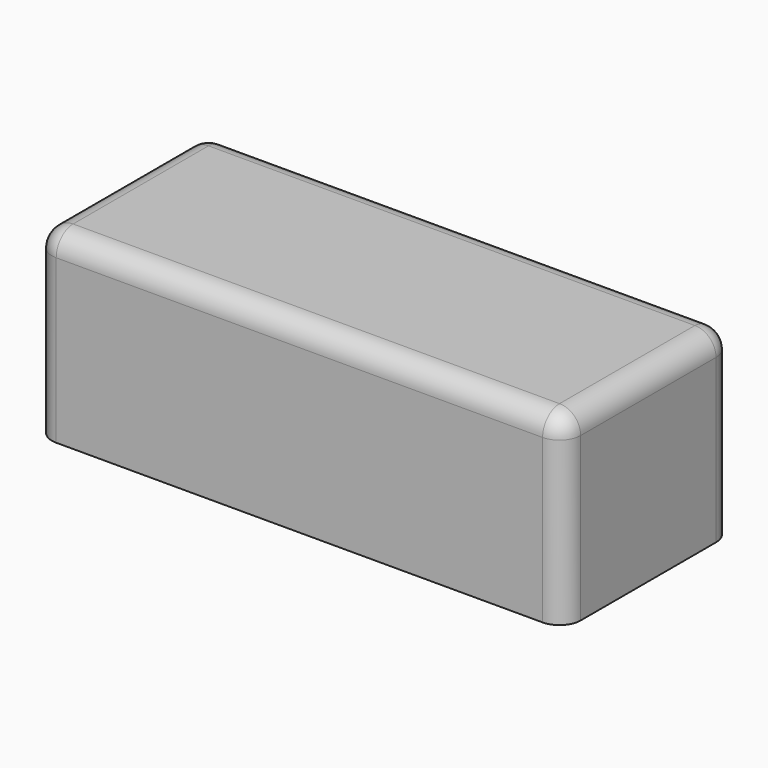
from build123d import *

# Parameters (mm, degrees)
F0_W         = 25
F0_H         = 10
F1_DEPTH     = 8
F2_W         = 25
F2_H         = 10
F3_DEPTH     = 0.7
F4_R         = 1
F5_T1_DEPTH  = 10.2
F5_S5_W      = 1
F5_S5_H      = 1
F5_T6_DEPTH  = 1
F6_T1_DEPTH  = 10.2
F6_S5_W      = 1
F6_S5_H      = 1
F6_T6_DEPTH  = 1
F6_S11_W     = 1
F6_S11_H     = 1
F6_T12_DEPTH = 1
F6_S17_W     = 1
F6_S17_H     = 1
F6_T18_DEPTH = 1


# Not quite as in the source:
# - a fillet or chamfer that OpenCascade refuses, or shapes differently, is made with other operations: its cross-section is extruded or revolved along the edge and cut away or added


with BuildPart() as f1:
    # F0 (on Top) → F1 (new body)
    with BuildSketch(Plane.XY):
        Rectangle(F0_W, F0_H)
        Polygon((-10, 2.45), (10, 2.45), (10, -2.45), (10, -3.65), (6.8, -3.65), (6.8, -2.45), (-6.8, -2.45), (-6.8, -3.65), (-10, -3.65), (-10, -2.45), align=None, mode=Mode.SUBTRACT)
    extrude(amount=F1_DEPTH)

    # F2 (on face) → F3 (join)
    with BuildSketch(Plane.XY.offset(8)):
        Rectangle(F2_W, F2_H)
    extrude(amount=F3_DEPTH)

    # F4
    f4_edges = [f1.edges().sort_by_distance(p)[0] for p in [
        (0, 5, 8.7),
        (-12.5, 0, 8.7),
        (0, -5, 8.7),
        (12.5, 0, 8.7),
    ]]
    fillet(f4_edges, radius=F4_R)

    # F5: fillet of radius 1 on 1 edges, made by hand

    # F5_s2 → F5_t1 (cut)
    with BuildSketch(Plane.XY.offset(-2.5)):
        with BuildLine():
            ThreePointArc((12.5, 4), (12.2071067812, 4.7071067812), (11.5, 5))
            Line((11.5, 5), (12.5, 5))
            Line((12.5, 5), (12.5, 4))
        make_face()
    extrude(amount=F5_T1_DEPTH, mode=Mode.SUBTRACT)


with BuildPart() as f5_tool4:
    # F5_s5 → F5_t6 (new body)
    with BuildSketch(Plane.YZ.offset(11.5)):
        with Locations((4.5, 8.2)):
            Rectangle(F5_S5_W, F5_S5_H)
    extrude(amount=F5_T6_DEPTH)

    # F5_s7 → F5_t8 (revolve, cut)
    with BuildSketch(Plane(origin=(11.5, 4, 7.7), x_dir=(0, -0.7071067812, -0.7071067812), z_dir=(0, -0.7071067812, 0.7071067812))):
        with BuildLine():
            ThreePointArc((0, -1), (1, 0), (0, 1))
            Line((0, 1), (0, -1))
        make_face()
    revolve(axis=Axis((11.5, 4, 7.7), (1, 0, 0)), mode=Mode.SUBTRACT)


with BuildPart() as f1_1:
    add(f1.part)

    # F5_t3: cut F5_tool4
    add(f5_tool4.part, mode=Mode.SUBTRACT)

    # F6: fillet of radius 1 on 3 edges, made by hand

    # F6_s2 → F6_t1 (cut)
    with BuildSketch(Plane.XY.offset(-2.5)):
        with BuildLine():
            ThreePointArc((-12.5, 4), (-12.2071067812, 4.7071067812), (-11.5, 5))
            Line((-11.5, 5), (-12.5, 5))
            Line((-12.5, 5), (-12.5, 4))
        make_face()
        with BuildLine():
            ThreePointArc((11.5, -5), (12.2071067812, -4.7071067812), (12.5, -4))
            Line((12.5, -4), (12.5, -5))
            Line((12.5, -5), (11.5, -5))
        make_face()
        with BuildLine():
            ThreePointArc((-11.5, -5), (-12.2071067812, -4.7071067812), (-12.5, -4))
            Line((-12.5, -4), (-12.5, -5))
            Line((-12.5, -5), (-11.5, -5))
        make_face()
    extrude(amount=F6_T1_DEPTH, mode=Mode.SUBTRACT)


with BuildPart() as f6_tool4:
    # F6_s5 → F6_t6 (new body)
    with BuildSketch(Plane.XZ.offset(4)):
        with Locations((-12, 8.2)):
            Rectangle(F6_S5_W, F6_S5_H)
    extrude(amount=F6_T6_DEPTH)

    # F6_s7 → F6_t8 (revolve, cut)
    with BuildSketch(Plane(origin=(-11.5, -4, 7.7), x_dir=(0.7071067812, 0, -0.7071067812), z_dir=(-0.7071067812, 0, -0.7071067812))):
        with BuildLine():
            ThreePointArc((0, -1), (1, 0), (0, 1))
            Line((0, 1), (0, -1))
        make_face()
    revolve(axis=Axis((-11.5, -4, 7.7), (0, -1, 0)), mode=Mode.SUBTRACT)


with BuildPart() as f1_2:
    add(f1_1.part)

    # F6_t3: cut F6_tool4
    add(f6_tool4.part, mode=Mode.SUBTRACT)


with BuildPart() as f6_tool10:
    # F6_s11 → F6_t12 (new body)
    with BuildSketch(Plane.XZ.offset(4)):
        with Locations((12, 8.2)):
            Rectangle(F6_S11_W, F6_S11_H)
    extrude(amount=F6_T12_DEPTH)

    # F6_s13 → F6_t14 (revolve, cut)
    with BuildSketch(Plane(origin=(11.5, -4, 7.7), x_dir=(-0.7071067812, 0, -0.7071067812), z_dir=(-0.7071067812, 0, 0.7071067812))):
        with BuildLine():
            ThreePointArc((0, -1), (1, 0), (0, 1))
            Line((0, 1), (0, -1))
        make_face()
    revolve(axis=Axis((11.5, -4, 7.7), (0, -1, 0)), mode=Mode.SUBTRACT)


with BuildPart() as f1_3:
    add(f1_2.part)

    # F6_t9: cut F6_tool10
    add(f6_tool10.part, mode=Mode.SUBTRACT)


with BuildPart() as f6_tool16:
    # F6_s17 → F6_t18 (new body)
    with BuildSketch(Plane.YZ.offset(-11.5)):
        with Locations((4.5, 8.2)):
            Rectangle(F6_S17_W, F6_S17_H)
    extrude(amount=-F6_T18_DEPTH)

    # F6_s19 → F6_t20 (revolve, cut)
    with BuildSketch(Plane(origin=(-11.5, 4, 7.7), x_dir=(0, -0.7071067812, -0.7071067812), z_dir=(0, 0.7071067812, -0.7071067812))):
        with BuildLine():
            ThreePointArc((0, -1), (1, 0), (0, 1))
            Line((0, 1), (0, -1))
        make_face()
    revolve(axis=Axis((-11.5, 4, 7.7), (-1, 0, 0)), mode=Mode.SUBTRACT)


with BuildPart() as f1_4:
    add(f1_3.part)

    # F6_t15: cut F6_tool16
    add(f6_tool16.part, mode=Mode.SUBTRACT)


solid = f1_4.part
